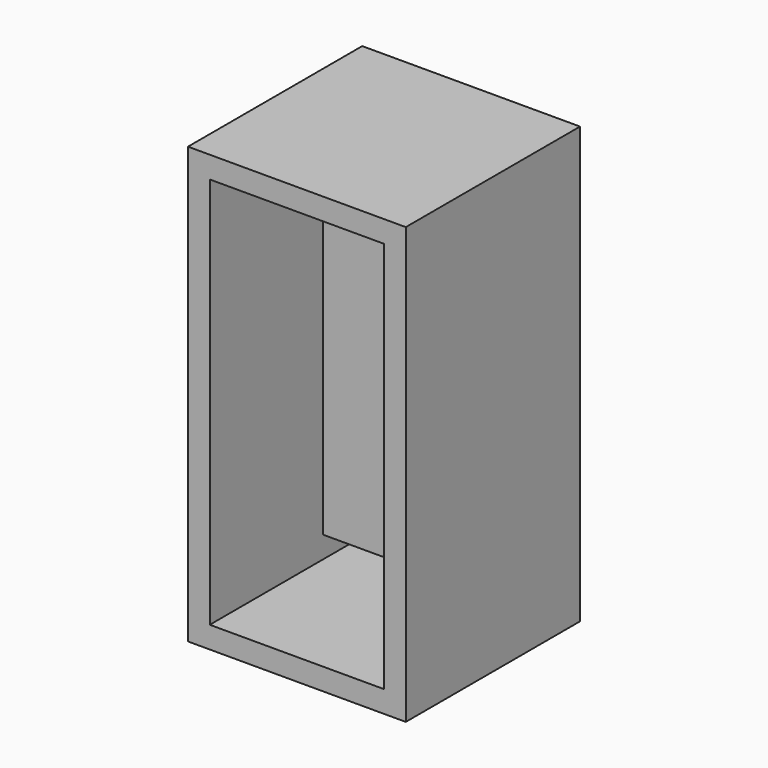
from build123d import *

# Parameters (mm, degrees)
F0_W          = 10
F0_H          = 20
F0_W_2        = 8
F0_H_2        = 18
F1_DEPTH      = 10
F2_W          = 2
F2_H          = 16
F3_DEPTH      = 10
F3_DEPTH_BACK = 0.01


with BuildPart() as f1:
    # F0 (on Front) → F1 (new body)
    with BuildSketch(Plane.XZ):
        with Locations((4, 9)):
            Rectangle(F0_W, F0_H)
        with Locations((4, 9)):
            Rectangle(F0_W_2, F0_H_2, mode=Mode.SUBTRACT)
    extrude(amount=F1_DEPTH)

    # F2 (on face) → F3 (join, two sides)
    with BuildSketch(Plane(origin=(-1, 0, 0), x_dir=(0, -1, 0), z_dir=(-1, 0, 0))) as f3_sk:
        with Locations((2.5, 9)):
            Rectangle(F2_W, F2_H)
    extrude(amount=-F3_DEPTH)
    extrude(f3_sk.sketch, amount=F3_DEPTH_BACK)


solid = f1.part
